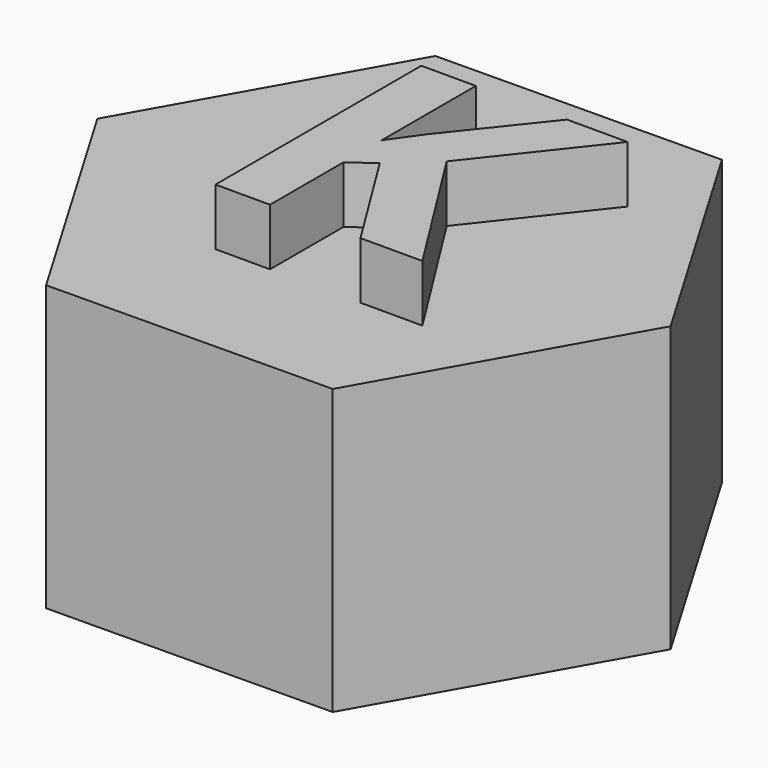
from build123d import *

# Parameters (mm, degrees)
F1_DEPTH     = 12.7
F2_TEXT_SIZE = 16.0924669924
F3_DEPTH     = 2.54


# Not quite as in the source:
# - Text() gives the source's letters only with a copy of the font that has no kerning and outlines rounded to 1/6400 em; it was checked with that copy


with BuildPart() as f1:
    # F0 (on Top) → F1 (new body)
    with BuildSketch(Plane.XY):
        Polygon((12.6993846473, 0.1250183213), (6.2414232815, 11.0604988776), (-6.4579613658, 10.9354805563), (-12.6993846473, -0.1250183213), (-6.2414232815, -11.0604988776), (6.4579613658, -10.9354805563), align=None)
    extrude(amount=F1_DEPTH)

    # F2 (on face) → F3 (join)
    with BuildSketch(Plane.XY.offset(12.7)):
        with Locations((-4.7755478881, -5.2452743985)):
            Text('K', F2_TEXT_SIZE, font='Open Sans', font_style=FontStyle.BOLD, text_align=(TextAlign.LEFT, TextAlign.BOTTOM))
    extrude(amount=F3_DEPTH)


solid = f1.part
